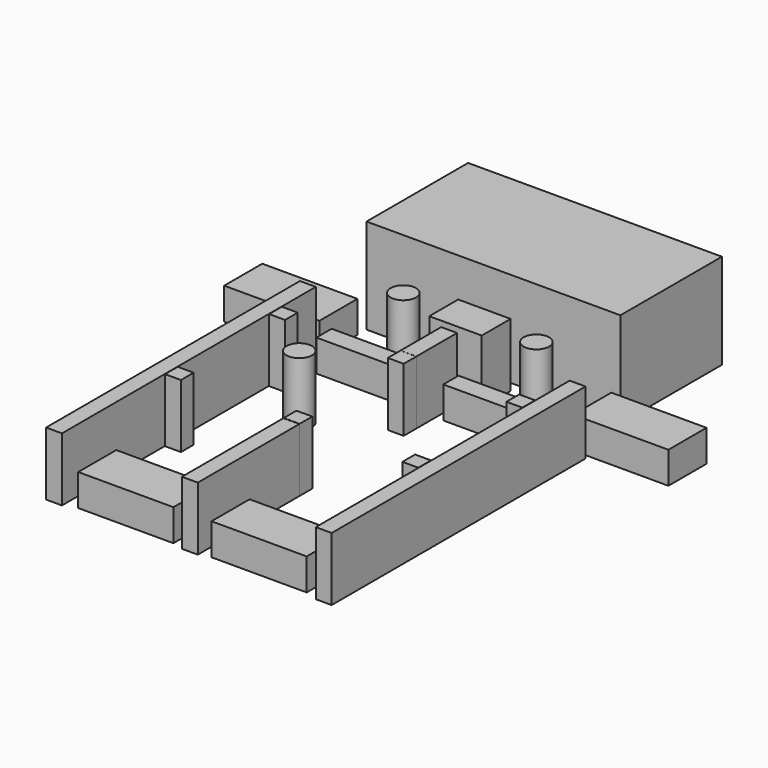
from build123d import *

# Parameters (mm, degrees)
F0_W      = 101.6
F0_H      = 50.8
F1_DEPTH  = 38.1
F2_W      = 38.1
F2_H      = 7.6261752665
F3_DEPTH  = 12.7
F4_W      = 6.35
F4_H      = 20.32
F5_DEPTH  = 25.4
F6_W      = 6.35
F6_H      = 127
F7_DEPTH  = 25.4
F8_W      = 3.175
F8_H      = 6.35
F9_DEPTH  = 25.4
F8_W_2    = 6.35
F10_W     = 6.35
F10_H     = 50.8
F12_DEPTH = 25.4
F13_W     = 38.1
F13_H     = 19.05
F14_DEPTH = 12.7
F15_R     = 5.08
F16_DEPTH = 25.4
F17_W     = 20.9910012782
F17_H     = 14.4560653716
F18_DEPTH = 25.4


# Not quite as in the source:
# - the program builds the solid bodies; features that only make, move or delete a surface that nothing else refers to are left out


with BuildPart() as f1:
    # F0 (on Top) → F1 (new body)
    with BuildSketch(Plane.XY):
        Rectangle(F0_W, F0_H)
    extrude(amount=F1_DEPTH)


with BuildPart() as f3:
    # F2 (on Top) → F3 (new body)
    with BuildSketch(Plane.XY):
        with Locations((-25.4, -54.6130876333)):
            Rectangle(F2_W, F2_H)
    extrude(amount=F3_DEPTH)


with BuildPart() as f3b:
    # F2 (on Top) → F3, piece 2 (new body)
    with BuildSketch(Plane.XY):
        with Locations((25.4, -54.6130876333)):
            Rectangle(F2_W, F2_H)
    extrude(amount=F3_DEPTH)


with BuildPart() as f5:
    # F4 (on Top) → F5 (new body)
    with BuildSketch(Plane.XY):
        with Locations((0, -57.74644104)):
            Rectangle(F4_W, F4_H)
    extrude(amount=F5_DEPTH)


with BuildPart() as f7:
    # F6 (on Top) → F7 (new body)
    with BuildSketch(Plane.XY):
        with Locations((-53.975, -114.3)):
            Rectangle(F6_W, F6_H)
    extrude(amount=F7_DEPTH)


with BuildPart() as f7b:
    # F6 (on Top) → F7, piece 2 (new body)
    with BuildSketch(Plane.XY):
        with Locations((53.975, -114.3)):
            Rectangle(F6_W, F6_H)
    extrude(amount=F7_DEPTH)


with BuildPart() as f9:
    # F8 (on Top) → F9 (new body)
    with BuildSketch(Plane.XY):
        with Locations((1.5875, -71.12)):
            Rectangle(F8_W, F8_H)
        with Locations((-1.5875, -71.12)):
            Rectangle(F8_W, F8_H)
    extrude(amount=F9_DEPTH)


with BuildPart() as f9b:
    # F8 (on Top) → F9, piece 2 (new body)
    with BuildSketch(Plane.XY):
        with Locations((47.498, -71.12)):
            Rectangle(F8_W_2, F8_H)
    extrude(amount=F9_DEPTH)


with BuildPart() as f9c:
    # F8 (on Top) → F9, piece 3 (new body)
    with BuildSketch(Plane.XY):
        with Locations((-47.498, -71.12)):
            Rectangle(F8_W_2, F8_H)
    extrude(amount=F9_DEPTH)


with BuildPart() as f9d:
    # F8 (on Top) → F9, piece 4 (new body)
    with BuildSketch(Plane.XY):
        with Locations((47.498, -123.19)):
            Rectangle(F8_W_2, F8_H)
    extrude(amount=F9_DEPTH)


with BuildPart() as f9e:
    # F8 (on Top) → F9, piece 5 (new body)
    with BuildSketch(Plane.XY):
        Polygon((0, -126.365), (3.175, -126.365), (3.175, -120.015), (0, -120.015), (-3.175, -120.015), (-3.175, -126.365), align=None)
    extrude(amount=F9_DEPTH)


with BuildPart() as f9f:
    # F8 (on Top) → F9, piece 6 (new body)
    with BuildSketch(Plane.XY):
        with Locations((-47.498, -123.19)):
            Rectangle(F8_W_2, F8_H)
    extrude(amount=F9_DEPTH)


with BuildPart() as f12:
    # F10 (on Top) → F12 (new body)
    with BuildSketch(Plane.XY):
        with Locations((0, -151.892)):
            Rectangle(F10_W, F10_H)
    extrude(amount=F12_DEPTH)


with BuildPart() as f14:
    # F13 (on Top) → F14 (new body)
    with BuildSketch(Plane.XY):
        with Locations((-69.85, -39.475132829)):
            Rectangle(F13_W, F13_H)
    extrude(amount=F14_DEPTH)


with BuildPart() as f14b:
    # F13 (on Top) → F14, piece 2 (new body)
    with BuildSketch(Plane.XY):
        with Locations((69.85, -39.475132829)):
            Rectangle(F13_W, F13_H)
    extrude(amount=F14_DEPTH)


with BuildPart() as f14c:
    # F13 (on Top) → F14, piece 3 (new body)
    with BuildSketch(Plane.XY):
        with Locations((26.67, -166.475132829)):
            Rectangle(F13_W, F13_H)
    extrude(amount=F14_DEPTH)


with BuildPart() as f14d:
    # F13 (on Top) → F14, piece 4 (new body)
    with BuildSketch(Plane.XY):
        with Locations((-26.67, -166.475132829)):
            Rectangle(F13_W, F13_H)
    extrude(amount=F14_DEPTH)


with BuildPart() as f16:
    # F15 (on Top) → F16 (new body)
    with BuildSketch(Plane.XY):
        with Locations((-27.8475936502, -87.757319212)):
            Circle(F15_R)
    extrude(amount=F16_DEPTH)


with BuildPart() as f16b:
    # F15 (on Top) → F16, piece 2 (new body)
    with BuildSketch(Plane.XY):
        with Locations((-26.9264988601, -36.8386283517)):
            Circle(F15_R)
    extrude(amount=F16_DEPTH)


with BuildPart() as f16c:
    # F15 (on Top) → F16, piece 3 (new body)
    with BuildSketch(Plane.XY):
        with Locations((26.3249278069, -36.8386283517)):
            Circle(F15_R)
    extrude(amount=F16_DEPTH)


with BuildPart() as f18:
    # F17 (on Top) → F18 (new body)
    with BuildSketch(Plane.XY):
        with Locations((-0.2067787573, -36.9087895378)):
            Rectangle(F17_W, F17_H)
    extrude(amount=F18_DEPTH)


solid = Compound([f1.part, f3.part, f3b.part, f5.part, f7.part, f7b.part, f9.part, f9b.part, f9c.part, f9d.part, f9e.part, f9f.part, f12.part, f14.part, f14b.part, f14c.part, f14d.part, f16.part, f16b.part, f16c.part, f18.part])
